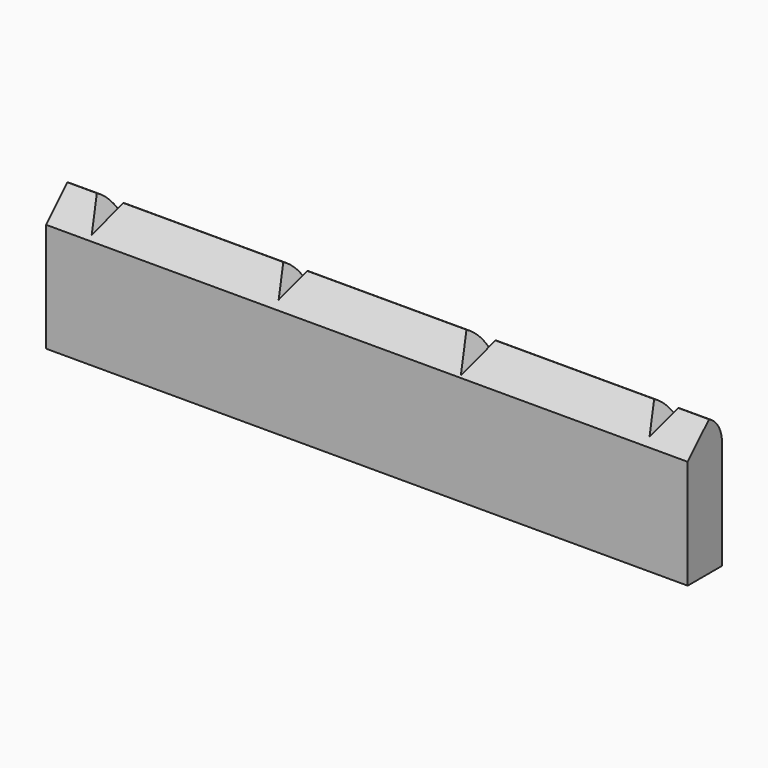
from build123d import *

# Parameters (mm, degrees)
F0_W        = 38.1
F0_H        = 2.54
F1_DEPTH    = 8.255
F3_R        = 1.778
F4_T1_DEPTH = 47.2449047052
F5_DEPTH    = 25.4


# Not quite as in the source:
# - a fillet or chamfer that OpenCascade refuses, or shapes differently, is made with other operations: its cross-section is extruded or revolved along the edge and cut away or added


with BuildPart() as f1:
    # F0 (on Top) → F1 (new body)
    with BuildSketch(Plane.XY):
        with Locations((0, 1.27)):
            Rectangle(F0_W, F0_H)
    extrude(amount=F1_DEPTH)

    # F3
    f3_edges = [f1.edges().sort_by_distance(p)[0] for p in [
        (0, 2.54, 8.255),
    ]]
    fillet(f3_edges, radius=F3_R)

    # F4: chamfer of 1.778 on 1 edges, made by hand

    # F4_s2 → F4_t1 (cut)
    with BuildSketch(Plane.YZ.offset(-23.6224523526)):
        Polygon((1.778, 8.255), (0, 6.477), (0, 8.255), align=None)
    extrude(amount=F4_T1_DEPTH, mode=Mode.SUBTRACT)

    # F2 (on face) → F5 (cut)
    with BuildSketch(Plane.XZ):
        Polygon((-16.51, 6.6902954744), (-15.6066174209, 8.255), (-17.4133825791, 8.255), align=None)
        Polygon((-4.6817409051, 8.255), (-6.3418590949, 8.255), (-5.5118, 6.8172954744), align=None)
        Polygon((6.4885060633, 8.255), (4.5350939367, 8.255), (5.5118, 6.5632954744), align=None)
        Polygon((17.3400590949, 8.255), (15.6799409051, 8.255), (16.51, 6.8172954744), align=None)
    extrude(amount=-F5_DEPTH, mode=Mode.SUBTRACT)


solid = f1.part
